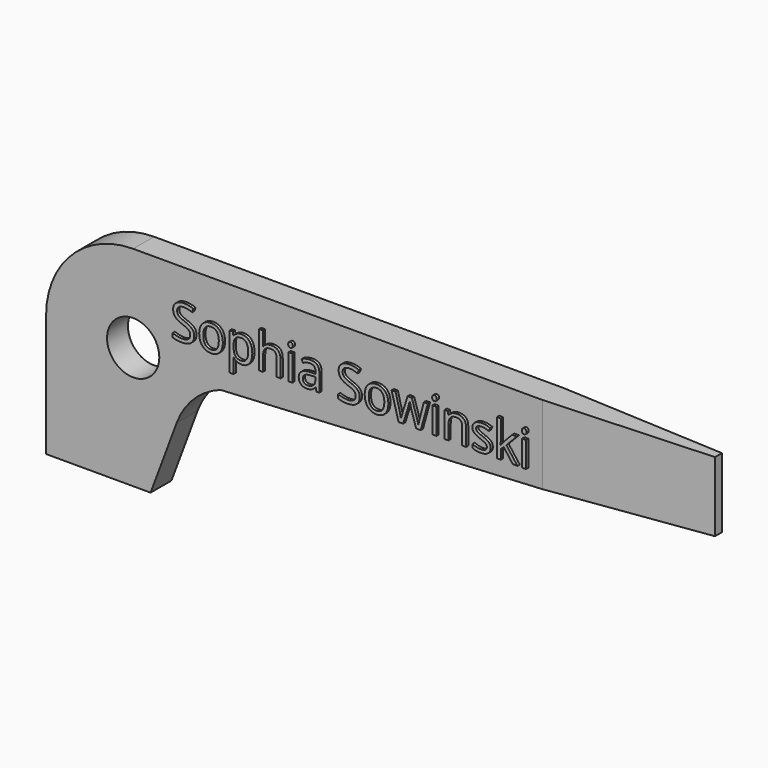
from build123d import *

# Parameters (mm, degrees)
F1_DEPTH     = 2.38125
F2_R         = 2.38125
F3_DEPTH     = 2.38225
F5_DEPTH     = 19.051
F6_TEXT_SIZE = 4.3739228406
F7_DEPTH     = 0.254


# Not quite as in the source:
# - Text() gives the source's letters only with a copy of the font that has no kerning and outlines rounded to 1/6400 em; it was checked with that copy


with BuildPart() as f1:
    # F0 (on Front) → F1 (new body)
    with BuildSketch(Plane.XZ):
        with BuildLine():
            Line((60.325, 19.05), (7.9375, 19.05))
            ThreePointArc((7.9375, 19.05), (2.3248399243, 16.7251600757), (0, 11.1125))
            Line((0, 11.1125), (0, 0))
            Line((0, 0), (9.525, 0))
            Line((9.525, 0), (11.906379987, 6.3821209389))
            ThreePointArc((11.906379987, 6.3821209389), (13.4661521943, 8.7911448047), (15.8957351173, 10.3186958333))
            Line((15.8957351173, 10.3186958333), (60.325, 12.7))
            Line((60.325, 12.7), (60.325, 19.05))
        make_face()
    extrude(amount=F1_DEPTH)

    # F2 (on face) → F3 (cut, through all)
    with BuildSketch(Plane.XZ.offset(2.38125)):
        with Locations((7.9375, 11.1125)):
            Circle(F2_R)
    extrude(amount=-F3_DEPTH, mode=Mode.SUBTRACT)

    # F4 (on face) → F5 (cut, through all)
    with BuildSketch(Plane.XY.offset(19.05)):
        Polygon((60.325, 0), (45.2374, 0), (60.325, -0.79375), align=None)
        Polygon((60.325, -2.38125), (60.325, -1.5875), (45.2374, -2.38125), align=None)
    extrude(amount=-F5_DEPTH, mode=Mode.SUBTRACT)

    # F6 (on face) → F7 (join)
    with BuildSketch(Plane.XZ.offset(2.38125)):
        with Locations((11.5143563598, 13.1873795763)):
            Text('Sophia Sowinski', F6_TEXT_SIZE, font='Open Sans', text_align=(TextAlign.LEFT, TextAlign.BOTTOM))
    extrude(amount=F7_DEPTH)


solid = f1.part
